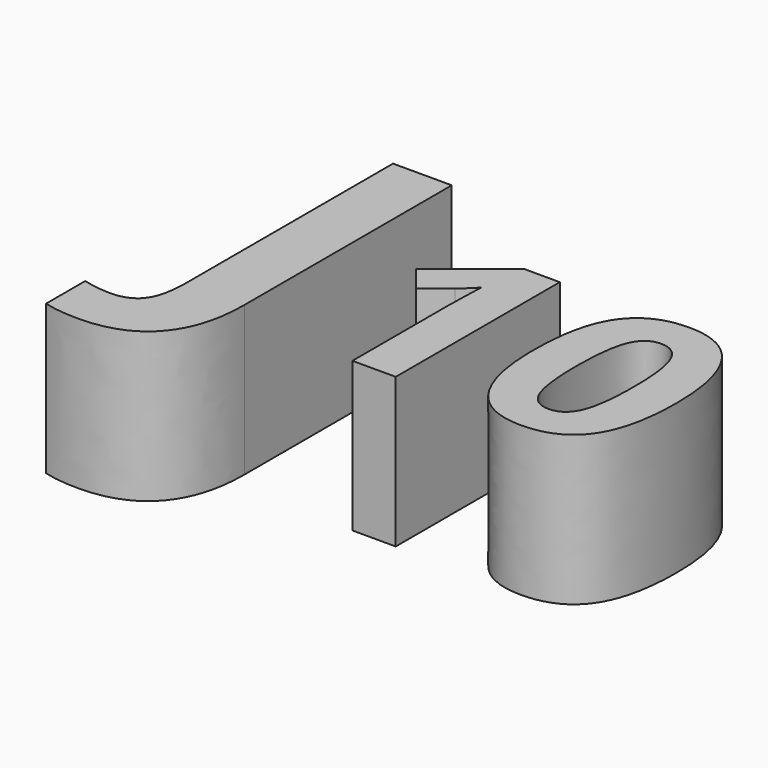
from build123d import *

# Parameters (mm, degrees)
F0_TEXT_SIZE   = 65.9505034693
F0_TEXT_SIZE_2 = 48.844233
F1_DEPTH       = 25.4
F2_DEPTH       = 25.4
F3_DEPTH       = 25.4


# Not quite as in the source:
# - Text() gives the source's letters only with a copy of the font that has no kerning and outlines rounded to 1/6400 em; it was checked with that copy


with BuildPart() as f1:
    # F0 (on Top) → F1 (new body)
    with BuildSketch(Plane.XY):
        with Locations((-49.2796599865, 14.5718287677)):
            Text('J', F0_TEXT_SIZE, font='Open Sans', font_style=FontStyle.BOLD, text_align=(TextAlign.LEFT, TextAlign.BOTTOM))
        with Locations((-24.9441028573, 13.9969848096)):
            Text('10', F0_TEXT_SIZE_2, font='Open Sans', font_style=FontStyle.BOLD, text_align=(TextAlign.LEFT, TextAlign.BOTTOM))
    extrude(amount=F1_DEPTH)


with BuildPart() as f2:
    # F0 (on Top) → F2 (new body)
    with BuildSketch(Plane.XY):
        with Locations((-49.2796599865, 14.5718287677)):
            Text('J', F0_TEXT_SIZE, font='Open Sans', font_style=FontStyle.BOLD, text_align=(TextAlign.LEFT, TextAlign.BOTTOM))
        with Locations((-24.9441028573, 13.9969848096)):
            Text('10', F0_TEXT_SIZE_2, font='Open Sans', font_style=FontStyle.BOLD, text_align=(TextAlign.LEFT, TextAlign.BOTTOM))
    extrude(amount=F2_DEPTH)


with BuildPart() as f3:
    # F0 (on Top) → F3 (new body)
    with BuildSketch(Plane.XY):
        with Locations((-49.2796599865, 14.5718287677)):
            Text('J', F0_TEXT_SIZE, font='Open Sans', font_style=FontStyle.BOLD, text_align=(TextAlign.LEFT, TextAlign.BOTTOM))
        with Locations((-24.9441028573, 13.9969848096)):
            Text('10', F0_TEXT_SIZE_2, font='Open Sans', font_style=FontStyle.BOLD, text_align=(TextAlign.LEFT, TextAlign.BOTTOM))
    extrude(amount=F3_DEPTH)


solid = Compound([f1.part, f2.part, f3.part])
